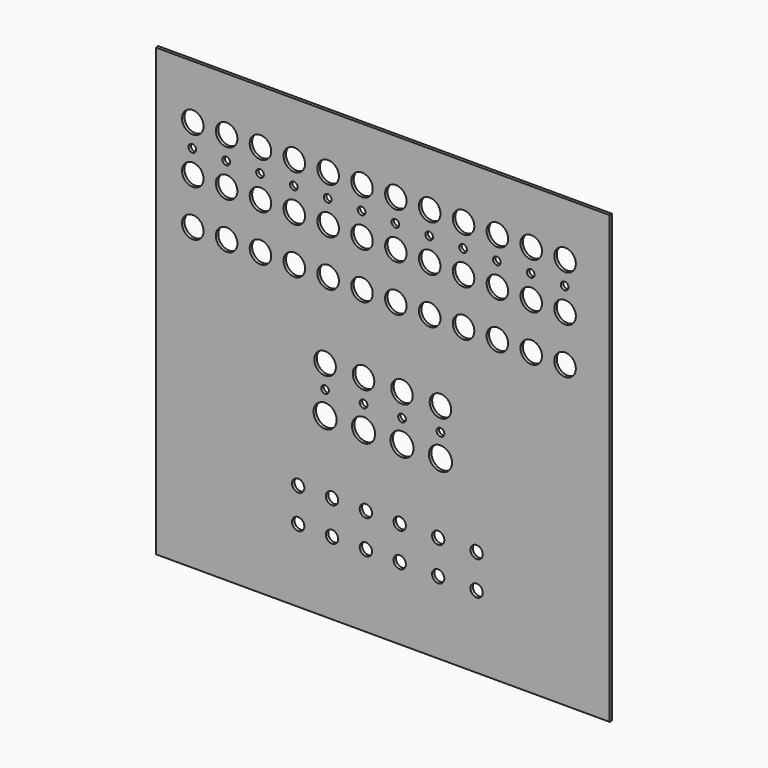
from build123d import *

# Parameters (mm, degrees)
F0_W      = 295
F0_H      = 290
F1_DEPTH  = 2
F3_DEPTH  = 25
F4_DEPTH  = 25
F6_DEPTH  = 25
F8_DEPTH  = 25
F9_R      = 7.5
F9_R_2    = 7
F9_R_3    = 2.5
F10_DEPTH = 25
F11_W     = 295
F11_H     = 290
F11_R     = 4
F11_R_2   = 7.5
F11_R_3   = 2.5
F11_R_4   = 7
F12_DEPTH = 2


# Not quite as in the source:
# - a feature names something its author has since deleted; it is built from what else it names


with BuildPart() as f1:
    # F0 (on Front) → F1 (new body)
    with BuildSketch(Plane.XZ):
        Rectangle(F0_W, F0_H)
    extrude(amount=-F1_DEPTH)

    # F2 (on face) → F3 (cut)
    with BuildSketch(Plane.XZ):
        with BuildLine():
            ThreePointArc((-116.5, 110), (-123.5, 117), (-130.5, 110))
            Line((-130.5, 110), (-116.5, 110))
        make_face()
        with BuildLine():
            Line((-116.5, 110), (-130.5, 110))
            ThreePointArc((-130.5, 110), (-123.5, 103), (-116.5, 110))
        make_face()
    extrude(amount=-F3_DEPTH, mode=Mode.SUBTRACT)

    # F2 (on face) → F4 (cut)
    with BuildSketch(Plane.XZ):
        with BuildLine():
            ThreePointArc((-116.5, 110), (-123.5, 117), (-130.5, 110))
            Line((-130.5, 110), (-116.5, 110))
        make_face()
        with BuildLine():
            ThreePointArc((125.5, 110), (118.5, 117), (111.5, 110))
            Line((111.5, 110), (125.5, 110))
        make_face()
        with BuildLine():
            Line((125.5, 110), (111.5, 110))
            ThreePointArc((111.5, 110), (118.5, 103), (125.5, 110))
        make_face()
        with BuildLine():
            ThreePointArc((103.5, 110), (96.5, 117), (89.5, 110))
            Line((89.5, 110), (103.5, 110))
        make_face()
        with BuildLine():
            Line((103.5, 110), (89.5, 110))
            ThreePointArc((89.5, 110), (96.5, 103), (103.5, 110))
        make_face()
        with BuildLine():
            ThreePointArc((81.5, 110), (74.5, 117), (67.5, 110))
            Line((67.5, 110), (81.5, 110))
        make_face()
        with BuildLine():
            Line((81.5, 110), (67.5, 110))
            ThreePointArc((67.5, 110), (74.5, 103), (81.5, 110))
        make_face()
        with BuildLine():
            ThreePointArc((59.5, 110), (52.5, 117), (45.5, 110))
            Line((45.5, 110), (59.5, 110))
        make_face()
        with BuildLine():
            Line((59.5, 110), (45.5, 110))
            ThreePointArc((45.5, 110), (52.5, 103), (59.5, 110))
        make_face()
        with BuildLine():
            ThreePointArc((37.5, 110), (30.5, 117), (23.5, 110))
            Line((23.5, 110), (37.5, 110))
        make_face()
        with BuildLine():
            Line((37.5, 110), (23.5, 110))
            ThreePointArc((23.5, 110), (30.5, 103), (37.5, 110))
        make_face()
        with BuildLine():
            ThreePointArc((15.5, 110), (8.5, 117), (1.5, 110))
            Line((1.5, 110), (15.5, 110))
        make_face()
        with BuildLine():
            Line((15.5, 110), (1.5, 110))
            ThreePointArc((1.5, 110), (8.5, 103), (15.5, 110))
        make_face()
        with BuildLine():
            ThreePointArc((-6.5, 110), (-13.5, 117), (-20.5, 110))
            Line((-20.5, 110), (-6.5, 110))
        make_face()
        with BuildLine():
            Line((-6.5, 110), (-20.5, 110))
            ThreePointArc((-20.5, 110), (-13.5, 103), (-6.5, 110))
        make_face()
        with BuildLine():
            ThreePointArc((-28.5, 110), (-35.5, 117), (-42.5, 110))
            Line((-42.5, 110), (-28.5, 110))
        make_face()
        with BuildLine():
            Line((-28.5, 110), (-42.5, 110))
            ThreePointArc((-42.5, 110), (-35.5, 103), (-28.5, 110))
        make_face()
        with BuildLine():
            ThreePointArc((-50.5, 110), (-57.5, 117), (-64.5, 110))
            Line((-64.5, 110), (-50.5, 110))
        make_face()
        with BuildLine():
            Line((-50.5, 110), (-64.5, 110))
            ThreePointArc((-64.5, 110), (-57.5, 103), (-50.5, 110))
        make_face()
        with BuildLine():
            ThreePointArc((-72.5, 110), (-79.5, 117), (-86.5, 110))
            Line((-86.5, 110), (-72.5, 110))
        make_face()
        with BuildLine():
            Line((-72.5, 110), (-86.5, 110))
            ThreePointArc((-86.5, 110), (-79.5, 103), (-72.5, 110))
        make_face()
        with BuildLine():
            ThreePointArc((-94.5, 110), (-101.5, 117), (-108.5, 110))
            Line((-108.5, 110), (-94.5, 110))
        make_face()
        with BuildLine():
            Line((-94.5, 110), (-108.5, 110))
            ThreePointArc((-108.5, 110), (-101.5, 103), (-94.5, 110))
        make_face()
        with BuildLine():
            Line((-116.5, 110), (-130.5, 110))
            ThreePointArc((-130.5, 110), (-123.5, 103), (-116.5, 110))
        make_face()
    extrude(amount=-F4_DEPTH, mode=Mode.SUBTRACT)

    # F5 (on face) → F6 (cut)
    with BuildSketch(Plane.XZ):
        with BuildLine():
            ThreePointArc((-116.5, 80), (-123.5, 87), (-130.5, 80))
            Line((-130.5, 80), (-116.5, 80))
        make_face()
        with BuildLine():
            Line((-116.5, 80), (-130.5, 80))
            ThreePointArc((-130.5, 80), (-123.5, 73), (-116.5, 80))
        make_face()
        with BuildLine():
            ThreePointArc((-116.5, 50), (-123.5, 57), (-130.5, 50))
            Line((-130.5, 50), (-116.5, 50))
        make_face()
        with BuildLine():
            Line((-116.5, 50), (-130.5, 50))
            ThreePointArc((-130.5, 50), (-123.5, 43), (-116.5, 50))
        make_face()
        with BuildLine():
            ThreePointArc((-94.5, 80), (-101.5, 87), (-108.5, 80))
            Line((-108.5, 80), (-94.5, 80))
        make_face()
        with BuildLine():
            Line((-94.5, 80), (-108.5, 80))
            ThreePointArc((-108.5, 80), (-101.5, 73), (-94.5, 80))
        make_face()
        with BuildLine():
            ThreePointArc((-72.5, 80), (-79.5, 87), (-86.5, 80))
            Line((-86.5, 80), (-72.5, 80))
        make_face()
        with BuildLine():
            Line((-72.5, 80), (-86.5, 80))
            ThreePointArc((-86.5, 80), (-79.5, 73), (-72.5, 80))
        make_face()
        with BuildLine():
            ThreePointArc((-50.5, 80), (-57.5, 87), (-64.5, 80))
            Line((-64.5, 80), (-50.5, 80))
        make_face()
        with BuildLine():
            Line((-50.5, 80), (-64.5, 80))
            ThreePointArc((-64.5, 80), (-57.5, 73), (-50.5, 80))
        make_face()
        with BuildLine():
            Line((-42.5, 80), (-28.5, 80))
            ThreePointArc((-28.5, 80), (-35.5, 87), (-42.5, 80))
        make_face()
        with BuildLine():
            ThreePointArc((-42.5, 80), (-35.5, 73), (-28.5, 80))
            Line((-28.5, 80), (-42.5, 80))
        make_face()
        with BuildLine():
            Line((-20.5, 80), (-6.5, 80))
            ThreePointArc((-6.5, 80), (-13.5, 87), (-20.5, 80))
        make_face()
        with BuildLine():
            ThreePointArc((-20.5, 80), (-13.5, 73), (-6.5, 80))
            Line((-6.5, 80), (-20.5, 80))
        make_face()
        with BuildLine():
            Line((1.5, 80), (15.5, 80))
            ThreePointArc((15.5, 80), (8.5, 87), (1.5, 80))
        make_face()
        with BuildLine():
            ThreePointArc((1.5, 80), (8.5, 73), (15.5, 80))
            Line((15.5, 80), (1.5, 80))
        make_face()
        with BuildLine():
            Line((23.5, 80), (37.5, 80))
            ThreePointArc((37.5, 80), (30.5, 87), (23.5, 80))
        make_face()
        with BuildLine():
            ThreePointArc((23.5, 80), (30.5, 73), (37.5, 80))
            Line((37.5, 80), (23.5, 80))
        make_face()
        with BuildLine():
            ThreePointArc((45.5, 80), (52.5, 73), (59.5, 80))
            Line((59.5, 80), (45.5, 80))
        make_face()
        with BuildLine():
            ThreePointArc((67.5, 80), (74.5, 73), (81.5, 80))
            Line((81.5, 80), (67.5, 80))
        make_face()
        with BuildLine():
            ThreePointArc((89.5, 80), (96.5, 73), (103.5, 80))
            Line((103.5, 80), (89.5, 80))
        make_face()
        with BuildLine():
            ThreePointArc((111.5, 80), (118.5, 73), (125.5, 80))
            Line((125.5, 80), (111.5, 80))
        make_face()
        with BuildLine():
            Line((111.5, 80), (125.5, 80))
            ThreePointArc((125.5, 80), (118.5, 87), (111.5, 80))
        make_face()
        with BuildLine():
            Line((89.5, 80), (103.5, 80))
            ThreePointArc((103.5, 80), (96.5, 87), (89.5, 80))
        make_face()
        with BuildLine():
            Line((67.5, 80), (81.5, 80))
            ThreePointArc((81.5, 80), (74.5, 87), (67.5, 80))
        make_face()
        with BuildLine():
            Line((45.5, 80), (59.5, 80))
            ThreePointArc((59.5, 80), (52.5, 87), (45.5, 80))
        make_face()
        with BuildLine():
            Line((111.5, 50), (125.5, 50))
            ThreePointArc((125.5, 50), (118.5, 57), (111.5, 50))
        make_face()
        with BuildLine():
            Line((89.5, 50), (103.5, 50))
            ThreePointArc((103.5, 50), (96.5, 57), (89.5, 50))
        make_face()
        with BuildLine():
            ThreePointArc((89.5, 50), (96.5, 43), (103.5, 50))
            Line((103.5, 50), (89.5, 50))
        make_face()
        with BuildLine():
            ThreePointArc((111.5, 50), (118.5, 43), (125.5, 50))
            Line((125.5, 50), (111.5, 50))
        make_face()
        with BuildLine():
            Line((67.5, 50), (81.5, 50))
            ThreePointArc((81.5, 50), (74.5, 57), (67.5, 50))
        make_face()
        with BuildLine():
            ThreePointArc((67.5, 50), (74.5, 43), (81.5, 50))
            Line((81.5, 50), (67.5, 50))
        make_face()
        with BuildLine():
            ThreePointArc((45.5, 50), (52.5, 43), (59.5, 50))
            Line((59.5, 50), (45.5, 50))
        make_face()
        with BuildLine():
            Line((45.5, 50), (59.5, 50))
            ThreePointArc((59.5, 50), (52.5, 57), (45.5, 50))
        make_face()
        with BuildLine():
            Line((23.5, 50), (37.5, 50))
            ThreePointArc((37.5, 50), (30.5, 57), (23.5, 50))
        make_face()
        with BuildLine():
            ThreePointArc((23.5, 50), (30.5, 43), (37.5, 50))
            Line((37.5, 50), (23.5, 50))
        make_face()
        with BuildLine():
            Line((1.5, 50), (15.5, 50))
            ThreePointArc((15.5, 50), (8.5, 57), (1.5, 50))
        make_face()
        with BuildLine():
            ThreePointArc((1.5, 50), (8.5, 43), (15.5, 50))
            Line((15.5, 50), (1.5, 50))
        make_face()
        with BuildLine():
            Line((-20.5, 50), (-6.5, 50))
            ThreePointArc((-6.5, 50), (-13.5, 57), (-20.5, 50))
        make_face()
        with BuildLine():
            ThreePointArc((-20.5, 50), (-13.5, 43), (-6.5, 50))
            Line((-6.5, 50), (-20.5, 50))
        make_face()
        with BuildLine():
            ThreePointArc((-28.5, 50), (-35.5, 57), (-42.5, 50))
            Line((-42.5, 50), (-28.5, 50))
        make_face()
        with BuildLine():
            Line((-28.5, 50), (-42.5, 50))
            ThreePointArc((-42.5, 50), (-35.5, 43), (-28.5, 50))
        make_face()
        with BuildLine():
            Line((-50.5, 50), (-64.5, 50))
            ThreePointArc((-64.5, 50), (-57.5, 43), (-50.5, 50))
        make_face()
        with BuildLine():
            ThreePointArc((-72.5, 50), (-79.5, 57), (-86.5, 50))
            Line((-86.5, 50), (-72.5, 50))
        make_face()
        with BuildLine():
            Line((-72.5, 50), (-86.5, 50))
            ThreePointArc((-86.5, 50), (-79.5, 43), (-72.5, 50))
        make_face()
        with BuildLine():
            Line((-94.5, 50), (-108.5, 50))
            ThreePointArc((-108.5, 50), (-101.5, 43), (-94.5, 50))
        make_face()
        with BuildLine():
            ThreePointArc((-50.5, 50), (-57.5, 57), (-64.5, 50))
            Line((-64.5, 50), (-50.5, 50))
        make_face()
        with BuildLine():
            ThreePointArc((-94.5, 50), (-101.5, 57), (-108.5, 50))
            Line((-108.5, 50), (-94.5, 50))
        make_face()
    extrude(amount=-F6_DEPTH, mode=Mode.SUBTRACT)

    # F7 (on face) → F8 (cut)
    with BuildSketch(Plane.XZ):
        with BuildLine():
            ThreePointArc((-126.3082945347, 95), (-123.8082945347, 92.5), (-121.3082945347, 95))
            Line((-121.3082945347, 95), (-126.3082945347, 95))
        make_face()
        with BuildLine():
            Line((-126.3082945347, 95), (-121.3082945347, 95))
            ThreePointArc((-121.3082945347, 95), (-123.8082945347, 97.5), (-126.3082945347, 95))
        make_face()
        with BuildLine():
            ThreePointArc((-99.3082945347, 95), (-101.8082945347, 97.5), (-104.3082945347, 95))
            Line((-104.3082945347, 95), (-99.3082945347, 95))
        make_face()
        with BuildLine():
            Line((-99.3082945347, 95), (-104.3082945347, 95))
            ThreePointArc((-104.3082945347, 95), (-101.8082945347, 92.5), (-99.3082945347, 95))
        make_face()
        with BuildLine():
            Line((-77.3082945347, 95), (-82.3082945347, 95))
            ThreePointArc((-82.3082945347, 95), (-79.8082945347, 92.5), (-77.3082945347, 95))
        make_face()
        with BuildLine():
            ThreePointArc((-77.3082945347, 95), (-79.8082945347, 97.5), (-82.3082945347, 95))
            Line((-82.3082945347, 95), (-77.3082945347, 95))
        make_face()
        with BuildLine():
            ThreePointArc((-55.3082945347, 95), (-57.8082945347, 97.5), (-60.3082945347, 95))
            Line((-60.3082945347, 95), (-55.3082945347, 95))
        make_face()
        with BuildLine():
            Line((-55.3082945347, 95), (-60.3082945347, 95))
            ThreePointArc((-60.3082945347, 95), (-57.8082945347, 92.5), (-55.3082945347, 95))
        make_face()
        with BuildLine():
            ThreePointArc((-33.3082945347, 95), (-35.8082945347, 97.5), (-38.3082945347, 95))
            Line((-38.3082945347, 95), (-33.3082945347, 95))
        make_face()
        with BuildLine():
            Line((-33.3082945347, 95), (-38.3082945347, 95))
            ThreePointArc((-38.3082945347, 95), (-35.8082945347, 92.5), (-33.3082945347, 95))
        make_face()
        with BuildLine():
            ThreePointArc((-11.3082945347, 95), (-13.8082945347, 97.5), (-16.3082945347, 95))
            Line((-16.3082945347, 95), (-11.3082945347, 95))
        make_face()
        with BuildLine():
            Line((-11.3082945347, 95), (-16.3082945347, 95))
            ThreePointArc((-16.3082945347, 95), (-13.8082945347, 92.5), (-11.3082945347, 95))
        make_face()
        with BuildLine():
            ThreePointArc((10.6917054653, 95), (8.1917054653, 97.5), (5.6917054653, 95))
            Line((5.6917054653, 95), (10.6917054653, 95))
        make_face()
        with BuildLine():
            Line((10.6917054653, 95), (5.6917054653, 95))
            ThreePointArc((5.6917054653, 95), (8.1917054653, 92.5), (10.6917054653, 95))
        make_face()
        with BuildLine():
            ThreePointArc((32.6917054653, 95), (30.1917054653, 97.5), (27.6917054653, 95))
            Line((27.6917054653, 95), (32.6917054653, 95))
        make_face()
        with BuildLine():
            Line((32.6917054653, 95), (27.6917054653, 95))
            ThreePointArc((27.6917054653, 95), (30.1917054653, 92.5), (32.6917054653, 95))
        make_face()
        with BuildLine():
            Line((49.6917054653, 95), (54.6917054653, 95))
            ThreePointArc((54.6917054653, 95), (52.1917054653, 97.5), (49.6917054653, 95))
        make_face()
        with BuildLine():
            ThreePointArc((49.6917054653, 95), (52.1917054653, 92.5), (54.6917054653, 95))
            Line((54.6917054653, 95), (49.6917054653, 95))
        make_face()
        with BuildLine():
            Line((71.6917054653, 95), (76.6917054653, 95))
            ThreePointArc((76.6917054653, 95), (74.1917054653, 97.5), (71.6917054653, 95))
        make_face()
        with BuildLine():
            ThreePointArc((71.6917054653, 95), (74.1917054653, 92.5), (76.6917054653, 95))
            Line((76.6917054653, 95), (71.6917054653, 95))
        make_face()
        with BuildLine():
            Line((93.6917054653, 95), (98.6917054653, 95))
            ThreePointArc((98.6917054653, 95), (96.1917054653, 97.5), (93.6917054653, 95))
        make_face()
        with BuildLine():
            ThreePointArc((93.6917054653, 95), (96.1917054653, 92.5), (98.6917054653, 95))
            Line((98.6917054653, 95), (93.6917054653, 95))
        make_face()
        with BuildLine():
            Line((115.6917054653, 95), (120.6917054653, 95))
            ThreePointArc((120.6917054653, 95), (118.1917054653, 97.5), (115.6917054653, 95))
        make_face()
        with BuildLine():
            ThreePointArc((115.6917054653, 95), (118.1917054653, 92.5), (120.6917054653, 95))
            Line((120.6917054653, 95), (115.6917054653, 95))
        make_face()
    extrude(amount=-F8_DEPTH, mode=Mode.SUBTRACT)

    # F9 (on face) → F10 (cut)
    with BuildSketch(Plane.XZ):
        with Locations((-37.5, -30)):
            Circle(F9_R)
        with Locations((-37.5, 0)):
            Circle(F9_R_2)
        with Locations((12.5, 0)):
            Circle(F9_R_2)
        with Locations((37.5, -30)):
            Circle(F9_R)
        with Locations((37.5, 0)):
            Circle(F9_R_2)
        with Locations((12.5, -30)):
            Circle(F9_R)
        with Locations((-12.5, -30)):
            Circle(F9_R)
        with Locations((12.5, -15)):
            Circle(F9_R_3)
        with Locations((-12.5, -15)):
            Circle(F9_R_3)
        with Locations((-37.5, -15)):
            Circle(F9_R_3)
        with Locations((37.5, -15)):
            Circle(F9_R_3)
        with Locations((-12.5, 0)):
            Circle(F9_R_2)
    extrude(amount=-F10_DEPTH, mode=Mode.SUBTRACT)

    # F11 (on face) → F12 (intersect)
    with BuildSketch(Plane.XZ):
        Rectangle(F11_W, F11_H)
        with Locations((-54.9993150739, -97.6248317928)):
            Circle(F11_R, mode=Mode.SUBTRACT)
        with Locations((-54.9993150739, -75.6248317928)):
            Circle(F11_R, mode=Mode.SUBTRACT)
        with Locations((-32.9995433826, -97.7250591895)):
            Circle(F11_R, mode=Mode.SUBTRACT)
        with Locations((-10.9997716913, -97.8252865861)):
            Circle(F11_R, mode=Mode.SUBTRACT)
        with Locations((-32.9995433826, -75.7250591895)):
            Circle(F11_R, mode=Mode.SUBTRACT)
        with Locations((-10.9997716913, -75.8252865861)):
            Circle(F11_R, mode=Mode.SUBTRACT)
        with Locations((-37.5, -30)):
            Circle(F11_R_2, mode=Mode.SUBTRACT)
        with Locations((-37.5, -15)):
            Circle(F11_R_3, mode=Mode.SUBTRACT)
        with Locations((-12.5, -30)):
            Circle(F11_R_2, mode=Mode.SUBTRACT)
        with Locations((-12.5, -15)):
            Circle(F11_R_3, mode=Mode.SUBTRACT)
        with Locations((11, -97.9255139828)):
            Circle(F11_R, mode=Mode.SUBTRACT)
        with Locations((36, -97.9255139828)):
            Circle(F11_R, mode=Mode.SUBTRACT)
        with Locations((11, -75.9255139828)):
            Circle(F11_R, mode=Mode.SUBTRACT)
        with Locations((36, -75.9255139828)):
            Circle(F11_R, mode=Mode.SUBTRACT)
        with Locations((61, -97.9255139828)):
            Circle(F11_R, mode=Mode.SUBTRACT)
        with Locations((61, -75.9255139828)):
            Circle(F11_R, mode=Mode.SUBTRACT)
        with Locations((12.5, -30)):
            Circle(F11_R_2, mode=Mode.SUBTRACT)
        with Locations((12.5, -15)):
            Circle(F11_R_3, mode=Mode.SUBTRACT)
        with Locations((37.5, -30)):
            Circle(F11_R_2, mode=Mode.SUBTRACT)
        with Locations((37.5, -15)):
            Circle(F11_R_3, mode=Mode.SUBTRACT)
        with Locations((-123.5, 50)):
            Circle(F11_R_4, mode=Mode.SUBTRACT)
        with Locations((-101.5, 50)):
            Circle(F11_R_4, mode=Mode.SUBTRACT)
        with Locations((-79.5, 50)):
            Circle(F11_R_4, mode=Mode.SUBTRACT)
        with Locations((-37.5, 0)):
            Circle(F11_R_4, mode=Mode.SUBTRACT)
        with Locations((-12.5, 0)):
            Circle(F11_R_4, mode=Mode.SUBTRACT)
        with Locations((-57.5, 50)):
            Circle(F11_R_4, mode=Mode.SUBTRACT)
        with Locations((-35.5, 50)):
            Circle(F11_R_4, mode=Mode.SUBTRACT)
        with Locations((-13.5, 50)):
            Circle(F11_R_4, mode=Mode.SUBTRACT)
        with Locations((-123.5, 80)):
            Circle(F11_R_4, mode=Mode.SUBTRACT)
        with Locations((-123.8082945347, 95)):
            Circle(F11_R_3, mode=Mode.SUBTRACT)
        with Locations((-101.5, 80)):
            Circle(F11_R_4, mode=Mode.SUBTRACT)
        with Locations((-79.5, 80)):
            Circle(F11_R_4, mode=Mode.SUBTRACT)
        with Locations((-101.8082945347, 95)):
            Circle(F11_R_3, mode=Mode.SUBTRACT)
        with Locations((-79.8082945347, 95)):
            Circle(F11_R_3, mode=Mode.SUBTRACT)
        with Locations((-123.5, 110)):
            Circle(F11_R_4, mode=Mode.SUBTRACT)
        with Locations((-101.5, 110)):
            Circle(F11_R_4, mode=Mode.SUBTRACT)
        with Locations((-79.5, 110)):
            Circle(F11_R_4, mode=Mode.SUBTRACT)
        with Locations((-57.5, 80)):
            Circle(F11_R_4, mode=Mode.SUBTRACT)
        with Locations((-57.8082945347, 95)):
            Circle(F11_R_3, mode=Mode.SUBTRACT)
        with Locations((-35.5, 80)):
            Circle(F11_R_4, mode=Mode.SUBTRACT)
        with Locations((-13.5, 80)):
            Circle(F11_R_4, mode=Mode.SUBTRACT)
        with Locations((-35.8082945347, 95)):
            Circle(F11_R_3, mode=Mode.SUBTRACT)
        with Locations((-13.8082945347, 95)):
            Circle(F11_R_3, mode=Mode.SUBTRACT)
        with Locations((-57.5, 110)):
            Circle(F11_R_4, mode=Mode.SUBTRACT)
        with Locations((-35.5, 110)):
            Circle(F11_R_4, mode=Mode.SUBTRACT)
        with Locations((-13.5, 110)):
            Circle(F11_R_4, mode=Mode.SUBTRACT)
        with Locations((12.5, 0)):
            Circle(F11_R_4, mode=Mode.SUBTRACT)
        with Locations((37.5, 0)):
            Circle(F11_R_4, mode=Mode.SUBTRACT)
        with Locations((8.5, 50)):
            Circle(F11_R_4, mode=Mode.SUBTRACT)
        with Locations((30.5, 50)):
            Circle(F11_R_4, mode=Mode.SUBTRACT)
        with Locations((52.5, 50)):
            Circle(F11_R_4, mode=Mode.SUBTRACT)
        with Locations((74.5, 50)):
            Circle(F11_R_4, mode=Mode.SUBTRACT)
        with Locations((96.5, 50)):
            Circle(F11_R_4, mode=Mode.SUBTRACT)
        with Locations((118.5, 50)):
            Circle(F11_R_4, mode=Mode.SUBTRACT)
        with Locations((8.5, 80)):
            Circle(F11_R_4, mode=Mode.SUBTRACT)
        with Locations((30.5, 80)):
            Circle(F11_R_4, mode=Mode.SUBTRACT)
        with Locations((8.1917054653, 95)):
            Circle(F11_R_3, mode=Mode.SUBTRACT)
        with Locations((30.1917054653, 95)):
            Circle(F11_R_3, mode=Mode.SUBTRACT)
        with Locations((52.5, 80)):
            Circle(F11_R_4, mode=Mode.SUBTRACT)
        with Locations((52.1917054653, 95)):
            Circle(F11_R_3, mode=Mode.SUBTRACT)
        with Locations((8.5, 110)):
            Circle(F11_R_4, mode=Mode.SUBTRACT)
        with Locations((30.5, 110)):
            Circle(F11_R_4, mode=Mode.SUBTRACT)
        with Locations((52.5, 110)):
            Circle(F11_R_4, mode=Mode.SUBTRACT)
        with Locations((74.5, 80)):
            Circle(F11_R_4, mode=Mode.SUBTRACT)
        with Locations((96.5, 80)):
            Circle(F11_R_4, mode=Mode.SUBTRACT)
        with Locations((74.1917054653, 95)):
            Circle(F11_R_3, mode=Mode.SUBTRACT)
        with Locations((96.1917054653, 95)):
            Circle(F11_R_3, mode=Mode.SUBTRACT)
        with Locations((118.5, 80)):
            Circle(F11_R_4, mode=Mode.SUBTRACT)
        with Locations((118.1917054653, 95)):
            Circle(F11_R_3, mode=Mode.SUBTRACT)
        with Locations((74.5, 110)):
            Circle(F11_R_4, mode=Mode.SUBTRACT)
        with Locations((96.5, 110)):
            Circle(F11_R_4, mode=Mode.SUBTRACT)
        with Locations((118.5, 110)):
            Circle(F11_R_4, mode=Mode.SUBTRACT)
    extrude(amount=-F12_DEPTH, mode=Mode.INTERSECT)


solid = f1.part
